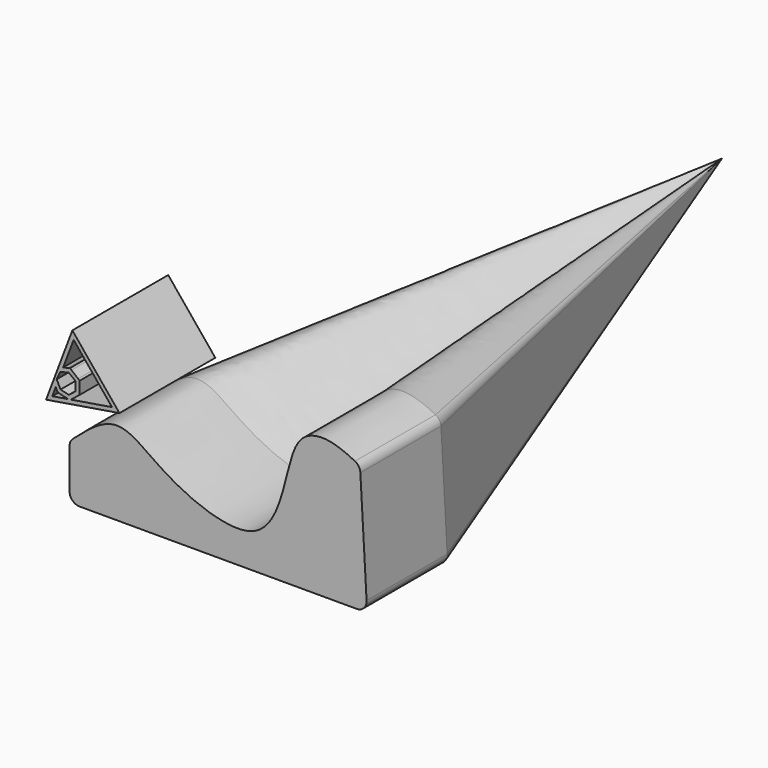
from build123d import *

# Parameters (mm, degrees)
F1_DEPTH    = 76.2
F3_DEPTH    = 147.066
F4_T        = 2.54
F4_T3_DEPTH = 81.28
F6_DEPTH    = 64.008


# Not quite as in the source:
# - a shell that OpenCascade refuses in one call is made with other operations: the cavity is built on its own and cut out


with BuildPart() as f1:
    # F0 (on Front) → F1 (new body)
    with BuildSketch(Plane.XZ):
        Polygon((-60.7324558319, 45.5212244649), (-77.4408412157, 1.2931352597), (-30.7839997113, 8.9372936636), align=None)
    extrude(amount=F1_DEPTH)

    # F2 (on face) → F3 (cut)
    with BuildSketch(Plane.XZ.offset(76.2)):
        Polygon((-58.5994124413, 12.1431014611), (-58.5994124413, 17.6589284913), (-62.9118596654, 21.0979903935), (-68.289393396, 19.8706034112), (-70.6826210522, 14.9010149762), (-68.289393396, 9.9314265412), (-62.9118596654, 8.7040395589), align=None)
    extrude(amount=-F3_DEPTH, mode=Mode.SUBTRACT)

    # F4: shell of thickness 2.54, made by hand


with BuildPart() as f4_core1:
    # F4_t2: copy of F1
    add(f1.part)

    # the walls: a layer under each face that stays
    f4_faces = [f4_core1.faces().sort_by_distance(p)[0] for p in [
        (-45.7582277716, -38.1, 27.2292590642),
        (-54.1124204635, -38.1, 5.1152144616),
        (-69.0866485238, -38.1, 23.4071798623),
        (-54.1124204635, 0, 23.4071798623),
        (-65.6006265307, -38.1, 9.31773305),
        (-60.7556360533, -38.1, 10.42357051),
        (-58.5994124413, -38.1, 14.9010149762),
        (-60.7556360533, -38.1, 19.3784594424),
        (-65.6006265307, -38.1, 20.4842969024),
        (-69.4860072241, -38.1, 17.3858091937),
        (-69.4860072241, -38.1, 12.4162207587),
    ]]
    thicken(f4_faces, amount=-F4_T, mode=Mode.SUBTRACT)

    # F4_s4 → F4_t3 (cut)
    with BuildSketch(Plane.XZ.offset(-2.54)):
        Polygon((-62.9220442746, 8.7486612475), (-63.4770628376, 6.2277226619), (-62.2845314719, 5.9555351597), (-61.3281955687, 6.7181875934), align=None)
        Polygon((-68.260856755, 9.9672103571), (-68.8545965682, 7.4551096442), (-70.0471279339, 7.7272971465), (-70.5778543204, 8.8293618438), align=None)
        Polygon((-58.6406490822, 12.1629599807), (-57.0157483445, 10.1572494956), (-56.0594124413, 10.9199019293), (-56.0594124413, 12.1431014611), align=None)
        Polygon((-58.6406490822, 17.6390699717), (-56.0594124413, 17.6589284913), (-56.0594124413, 18.8821280231), (-57.0157483445, 19.6447804568), align=None)
        Polygon((-62.9220442746, 21.0533687049), (-61.3281955687, 23.083842359), (-62.2845314719, 23.8464947927), (-63.4770628376, 23.5743072905), align=None)
        Polygon((-68.260856755, 19.8348195953), (-68.8545965682, 22.3469203082), (-70.0471279339, 22.0747328059), (-70.5778543204, 20.9726681086), align=None)
        Polygon((-70.6368518337, 14.9010149762), (-72.9710819767, 16.0030796736), (-73.5018083632, 14.9010149762), (-72.9710819767, 13.7989502788), align=None)
    extrude(amount=F4_T3_DEPTH, mode=Mode.SUBTRACT)


with BuildPart() as f1_1:
    add(f1.part)

    # what is left inside the walls is the cavity
    f4_cavity = [f4_core1.part.solids().sort_by_distance(p)[0] for p in [
        (-47.743308, -51.646667, 25.604226),
        (-68.404633, -51.646667, 5.373212),
    ]]
    add(f4_cavity, mode=Mode.SUBTRACT)


with BuildPart() as f6:
    # F5 (on Front) → F6 (new body)
    with BuildSketch(Plane.XZ):
        with BuildLine():
            add(Edge.make_bspline(
                [(-70.1527648421, -23.2108536477), (-60.6990565343, -14.7232992277), (-40.9831926516, 1.83381703), (-12.2629259812, -26.9568248212), (51.4022618375, -51.0895375253), (65.529569725, -2.8446328483), (71.6692230304, 26.1579596988), (90.6486190208, 30.8684291296), (103.5622151331, 25.4783434223), (109.2059325905, 22.5790402468)],
                knots=[0.0102259342, 0.0102259342, 0.0102259342, 0.0102259342, 0.1478911317, 0.299732983, 0.4877590798, 0.6455940504, 0.7791147117, 0.8809245501, 0.9804212447, 0.9804212447, 0.9804212447, 0.9804212447], degree=3))
            ThreePointArc((-70.1527648421, -23.2108536477), (-71.7097346741, -25.3489819727), (-72.2605809569, -27.9359331057))
            Line((-72.2605809569, -27.9359331057), (-72.2605809569, -53.3737758338))
            ThreePointArc((-72.2605809569, -53.3737758338), (-70.4007090175, -57.8639038944), (-65.9105809569, -59.7237758338))
            Line((-65.9105809569, -59.7237758338), (110.2651199851, -59.7237758338))
            ThreePointArc((110.2651199851, -59.7237758338), (114.8798030522, -57.7357937373), (116.6050664914, -53.0165947912))
            Line((116.6050664914, -53.0165947912), (112.6442364527, 17.2879498755))
            ThreePointArc((112.6442364527, 17.2879498755), (111.6288229621, 20.3908046946), (109.2059325905, 22.5790402468))
        make_face()
    extrude(amount=F6_DEPTH)

    # F6_face (on face) → F9 section 0
    with BuildSketch(Plane(origin=(34.7515553304, 0, -30.0784003182), x_dir=(1, 0, 0), z_dir=(0, 1, 0)), mode=Mode.PRIVATE) as f9_s0:
        with BuildLine():
            add(Edge.make_bspline(
                [(-104.9043201725, -6.8675466705), (-95.4506118647, -15.3551010905), (-75.734747982, -31.9122173482), (-47.0144813117, -3.121575497), (16.6507065071, 21.0111372071), (30.7780143945, -27.2337674699), (36.9176677, -56.236360017), (55.8970636904, -60.9468294478), (68.8106598027, -55.5567437405), (74.4543772601, -52.657440565)],
                knots=[0.0102259342, 0.0102259342, 0.0102259342, 0.0102259342, 0.1478911317, 0.299732983, 0.4877590798, 0.6455940504, 0.7791147117, 0.8809245501, 0.9804212447, 0.9804212447, 0.9804212447, 0.9804212447], degree=3))
            ThreePointArc((74.4543772601, -52.657440565), (76.8772676317, -50.4692050128), (77.8926811222, -47.3663501937))
            Line((77.8926811222, -47.3663501937), (81.8535111609, 22.938194473))
            ThreePointArc((81.8535111609, 22.938194473), (80.1282477218, 27.6573934191), (75.5135646546, 29.6453755157))
            Line((75.5135646546, 29.6453755157), (-100.6621362874, 29.6453755157))
            ThreePointArc((-100.6621362874, 29.6453755157), (-105.1522643479, 27.7855035762), (-107.0121362874, 23.2953755157))
            Line((-107.0121362874, 23.2953755157), (-107.0121362874, -2.1424672125))
            ThreePointArc((-107.0121362874, -2.1424672125), (-106.4612900045, -4.7294183455), (-104.9043201725, -6.8675466705))
        make_face()
    loft([f9_s0.sketch, Vertex(21.0942756385, 337.82, 0)])


solid = Compound([f1_1.part, f6.part])
